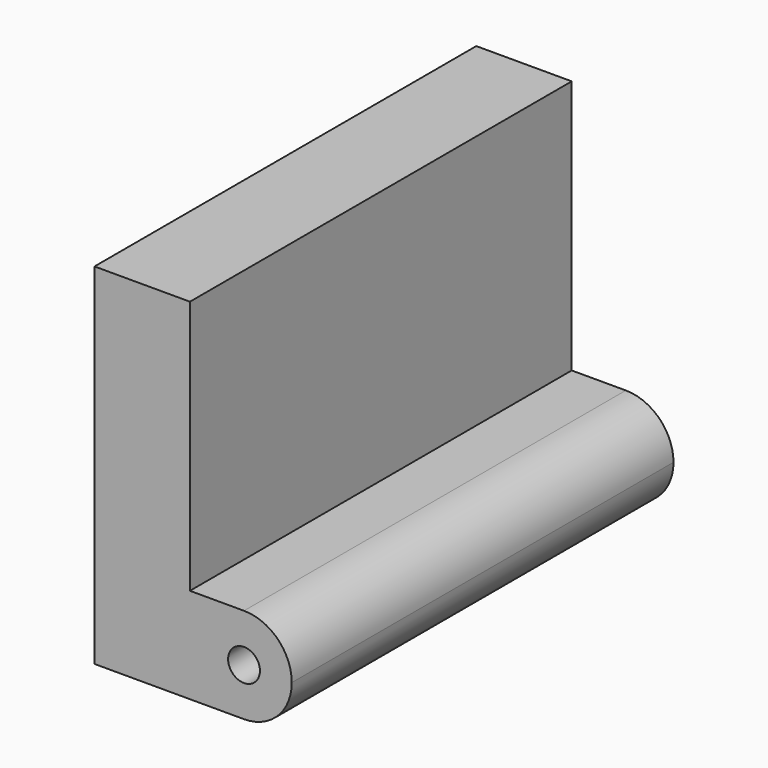
from build123d import *

# Parameters (mm, degrees)
F1_DEPTH = 95.25
F2_R     = 9.52499
F3_R     = 3.175
F4_DEPTH = 95.251


# Not quite as in the source:
# - a fillet or chamfer is up to 0.001 mm smaller than in the source, because OpenCascade refuses the exact size
# - a feature names something its author has since deleted; it is built from what else it names


with BuildPart() as f1:
    # F0 (on Front) → F1 (new body)
    with BuildSketch(Plane.XZ):
        Polygon((-12.472799319, 39.8380596402), (-31.522799319, 39.8380596402), (-31.522799319, -30.0119403598), (7.847200681, -30.0119403598), (7.847200681, -10.9619403598), (-12.472799319, -10.9619403598), align=None)
    extrude(amount=F1_DEPTH)

    # F2 (radius 9.525 in the source; OpenCascade refuses exactly that, so slightly less here)
    f2_edges = [f1.edges().sort_by_distance(p)[0] for p in [
        (7.847201, -47.625, -10.96194),
        (7.847201, -47.625, -30.01194),
    ]]
    fillet(f2_edges, radius=F2_R)

    # F3 (on face) → F4 (cut, through all)
    with BuildSketch(Plane.XZ.offset(95.25)):
        with Locations((-1.677799319, -20.4869403598)):
            Circle(F3_R)
    extrude(amount=-F4_DEPTH, mode=Mode.SUBTRACT)


solid = f1.part
